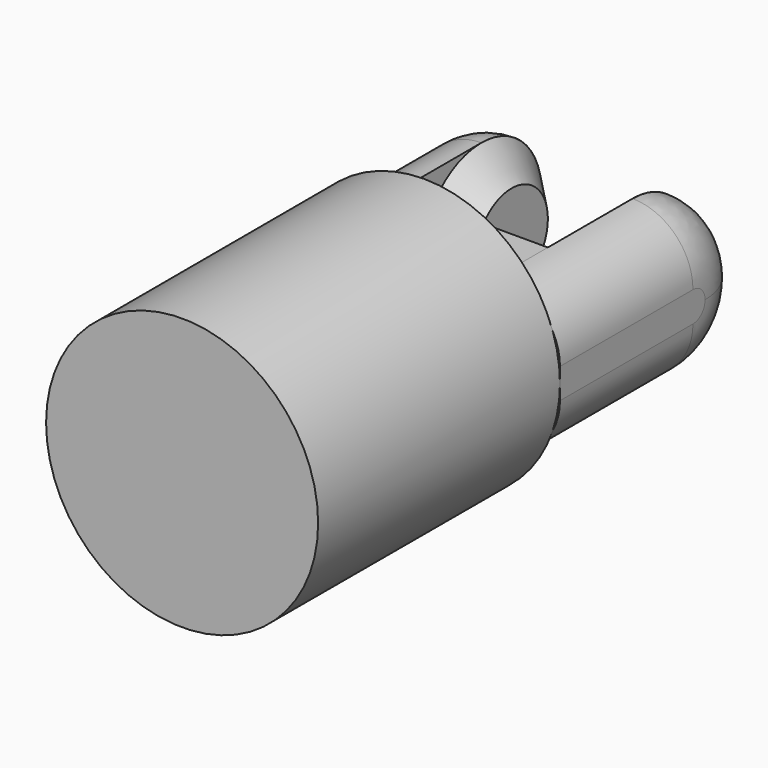
from build123d import *
from build123d import SkipClean  # not in build123d's __all__

# Parameters (mm, degrees)
F1_DEPTH      = 5
F2_R          = 2.5
F3_DEPTH      = 1
F4_SIZE       = 0.99999
F5_R          = 2.5
F6_DEPTH      = 1
F7_SIZE       = 0.99999
F8_R          = 2.4999
F9_R          = 4.5
F10_DEPTH     = 10
F11_T1_DEPTH  = 5.5001
F11_T3_DEPTH  = 0.0002
F11_T6_ANGLE  = 90
F11_T8_ANGLE  = 90
F11_T10_ANGLE = 90
F11_T12_ANGLE = 90


# Not quite as in the source:
# - a fillet or chamfer that OpenCascade refuses, or shapes differently, is made with other operations: its cross-section is extruded or revolved along the edge and cut away or added
# - a fillet or chamfer is up to 0.001 mm smaller than in the source, because OpenCascade refuses the exact size


with BuildPart() as f1:
    # F0 (on Top) → F1 (new body)
    with BuildSketch(Plane.XY):
        Polygon((15.446737438, 4.2690986316), (10.446737438, 4.2690986316), (10.446737438, 10.2690986316), (8.446737438, 10.2690986316), (8.446737438, 2.2690986316), (17.446737438, 2.2690986316), (17.446737438, 10.2690986316), (15.446737438, 10.2690986316), align=None)
    extrude(amount=F1_DEPTH)

    # F2 (on face) → F3 (join)
    with BuildSketch(Plane.YZ.offset(10.446737438)):
        with Locations((7.7690986316, 2.5)):
            Circle(F2_R)
    extrude(amount=F3_DEPTH)

    # F4 (size 1 in the source; OpenCascade refuses exactly that, so slightly less here)
    f4_edges = [f1.edges().sort_by_distance(p)[0] for p in [
        (11.446737, 5.269099, 2.5),
    ]]
    chamfer(f4_edges, length=F4_SIZE)

    # F5 (on face) → F6 (join)
    with BuildSketch(Plane(origin=(15.446737438, 0, 0), x_dir=(0, -1, 0), z_dir=(-1, 0, 0))):
        with Locations((-7.7690986316, 2.5)):
            Circle(F5_R)
    extrude(amount=F6_DEPTH)

    # F7 (size 1 in the source; OpenCascade refuses exactly that, so slightly less here)
    f7_edges = [f1.edges().sort_by_distance(p)[0] for p in [
        (14.446737, 10.269099, 2.5),
    ]]
    chamfer(f7_edges, length=F7_SIZE)

    # F8 (radius 2.5 in the source; OpenCascade refuses exactly that, so slightly less here)
    f8_edges = [f1.edges().sort_by_distance(p)[0] for p in [
        (16.446737, 10.269099, 5),
        (16.446737, 10.269099, 0),
        (9.446737, 10.269099, 5),
        (9.446737, 10.269099, 0),
    ]]
    fillet(f8_edges, radius=F8_R)

    # F9 (on face) → F10 (join)
    with BuildSketch(Plane.XZ.offset(-2.2690986316)):
        with Locations((12.946737438, 2.5)):
            Circle(F9_R)
    extrude(amount=F10_DEPTH)

    # F11: fillet of radius 2 on 4 edges, made by hand

    # F11_s2 → F11_t1 (cut)
    with BuildSketch(Plane.XZ.offset(-7.7691986316)):
        with BuildLine():
            ThreePointArc((8.446737438, 3), (9.0325238756, 4.4142135624), (10.446737438, 5))
            Line((10.446737438, 5), (8.446737438, 5))
            Line((8.446737438, 5), (8.446737438, 3))
        make_face()
        with BuildLine():
            ThreePointArc((10.446737438, 0), (9.0325238756, 0.5857864376), (8.446737438, 2))
            Line((8.446737438, 2), (8.446737438, 0))
            Line((8.446737438, 0), (10.446737438, 0))
        make_face()
        with BuildLine():
            ThreePointArc((15.446737438, 0), (16.8609510003, 0.5857864376), (17.446737438, 2))
            Line((17.446737438, 2), (17.446737438, 0))
            Line((17.446737438, 0), (15.446737438, 0))
        make_face()
        with BuildLine():
            ThreePointArc((17.446737438, 3), (16.8609510003, 4.4142135624), (15.446737438, 5))
            Line((15.446737438, 5), (17.446737438, 5))
            Line((17.446737438, 5), (17.446737438, 3))
        make_face()
    extrude(amount=F11_T1_DEPTH, mode=Mode.SUBTRACT)

    # F11_s4 → F11_t3 (cut)
    with BuildSketch(Plane.XY.offset(2.4999)):
        with BuildLine():
            ThreePointArc((15.446737438, 10.2690986316), (16.8609510003, 9.6833121939), (17.446737438, 8.2690986316))
            Line((17.446737438, 8.2690986316), (17.446737438, 10.2690986316))
            Line((17.446737438, 10.2690986316), (15.446737438, 10.2690986316))
        make_face()
        with BuildLine():
            ThreePointArc((8.446737438, 8.2690986316), (9.0325238756, 9.6833121939), (10.446737438, 10.2690986316))
            Line((10.446737438, 10.2690986316), (8.446737438, 10.2690986316))
            Line((8.446737438, 10.2690986316), (8.446737438, 8.2690986316))
        make_face()
    with SkipClean():  # cleaning this boolean's faces spoils the solid; the shape is the same uncleaned
        extrude(amount=F11_T3_DEPTH, mode=Mode.SUBTRACT)

    # F11_s5 → F11_t6 (revolve, cut)
    with BuildSketch(Plane.XZ.offset(-7.7691986316)):
        with BuildLine():
            ThreePointArc((17.446737438, 3), (16.8609510003, 4.4142135624), (15.446737438, 5))
            Line((15.446737438, 5), (17.446737438, 5))
            Line((17.446737438, 5), (17.446737438, 3))
        make_face()
    with SkipClean():  # cleaning this boolean's faces spoils the solid; the shape is the same uncleaned
        revolve(axis=Axis((17.446737438, 7.7691986316, 2.5001), (-1, 0, 0)), revolution_arc=F11_T6_ANGLE, mode=Mode.SUBTRACT)

    # F11_s7 → F11_t8 (revolve, cut)
    with BuildSketch(Plane.XZ.offset(-7.7691986316)):
        with BuildLine():
            ThreePointArc((15.446737438, 0), (16.8609510003, 0.5857864376), (17.446737438, 2))
            Line((17.446737438, 2), (17.446737438, 0))
            Line((17.446737438, 0), (15.446737438, 0))
        make_face()
    with SkipClean():  # cleaning this boolean's faces spoils the solid; the shape is the same uncleaned
        revolve(axis=Axis((17.446737438, 7.7691986316, 2.4999), (1, 0, 0)), revolution_arc=F11_T8_ANGLE, mode=Mode.SUBTRACT)

    # F11_s9 → F11_t10 (revolve, cut)
    with BuildSketch(Plane.XZ.offset(-7.7691986316)):
        with BuildLine():
            ThreePointArc((10.446737438, 0), (9.0325238756, 0.5857864376), (8.446737438, 2))
            Line((8.446737438, 2), (8.446737438, 0))
            Line((8.446737438, 0), (10.446737438, 0))
        make_face()
    revolve(axis=Axis((8.446737438, 7.7691986316, 2.4999), (1, 0, 0)), revolution_arc=F11_T10_ANGLE, mode=Mode.SUBTRACT)

    # F11_s11 → F11_t12 (revolve, cut)
    with BuildSketch(Plane.XZ.offset(-7.7691986316)):
        with BuildLine():
            ThreePointArc((8.446737438, 3), (9.0325238756, 4.4142135624), (10.446737438, 5))
            Line((10.446737438, 5), (8.446737438, 5))
            Line((8.446737438, 5), (8.446737438, 3))
        make_face()
    revolve(axis=Axis((8.446737438, 7.7691986316, 2.5001), (-1, 0, 0)), revolution_arc=F11_T12_ANGLE, mode=Mode.SUBTRACT)


solid = f1.part
